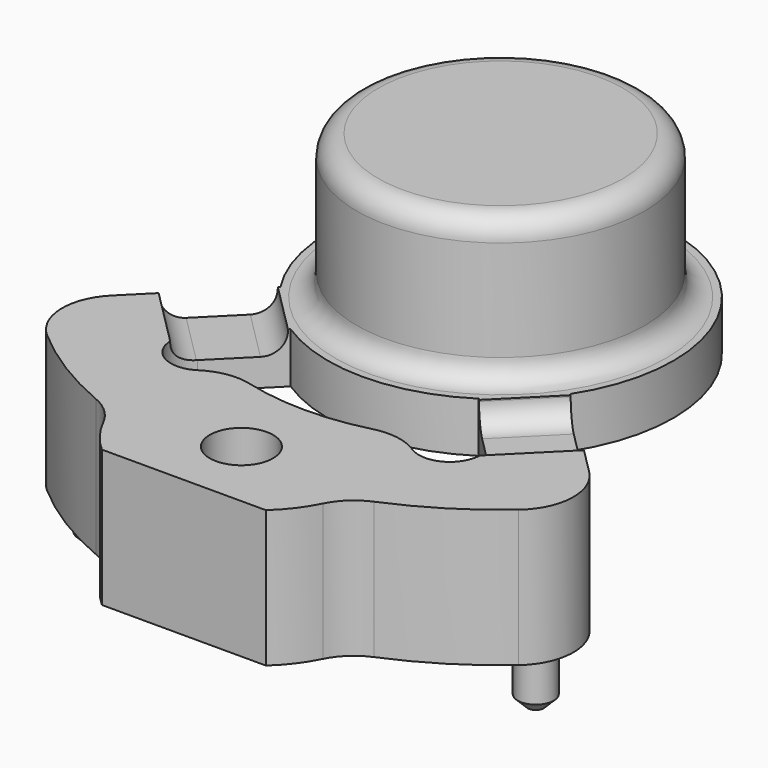
from build123d import *

# Parameters (mm, degrees)
F0_R      = 1.1
F1_DEPTH  = 4.75
F2_R      = 5
F3_DEPTH  = 5
F5_R      = 2
F7_DEPTH  = 0.8
F8_R      = 0.75
F9_R      = 9.5
F10_DEPTH = 3
F12_R     = 4.5172071506
F12_R_2   = 2.2672071506
F13_DEPTH = 3.7
F14_R     = 0.625
F15_DEPTH = 2
F16_SIZE  = 0.35


# Not quite as in the source:
# - a feature names something its author has since deleted; it is built from what else it names


with BuildPart() as f1:
    # F0 (on Top) → F1 (new body)
    with BuildSketch(Plane.XY):
        with BuildLine():
            Line((-5.0334316447, -3.2656646917), (-9.6784130262, -7.9106460732))
            ThreePointArc((-9.6784130262, -7.9106460732), (-7.1490584463, -10.2538267653), (-4.0757746589, -11.8168549509))
            ThreePointArc((-4.0757746589, -11.8168549509), (-3.593311946, -12.8676823003), (-2.8459674038, -13.75))
            Line((-2.8459674038, -13.75), (2.8459674038, -13.75))
            ThreePointArc((2.8459674038, -13.75), (3.593311946, -12.8676823003), (4.0757746589, -11.8168549509))
            ThreePointArc((4.0757746589, -11.8168549509), (7.1490584463, -10.2538267653), (9.6784130262, -7.9106460732))
            Line((9.6784130262, -7.9106460732), (5.0334316447, -3.2656646917))
            ThreePointArc((5.0334316447, -3.2656646917), (0, 6), (-5.0334316447, -3.2656646917))
        make_face()
        with Locations((0, -11.25)):
            Circle(F0_R, mode=Mode.SUBTRACT)
        with BuildLine():
            Line((-5.061459087, -6.82922604), (-3.2656646917, -5.0334316447))
            ThreePointArc((-3.2656646917, -5.0334316447), (0, -6), (3.2656646917, -5.0334316447))
            Line((3.2656646917, -5.0334316447), (5.061459087, -6.82922604))
            ThreePointArc((5.061459087, -6.82922604), (4.8326547168, -8.5179809488), (3.2656646917, -7.8480653995))
            ThreePointArc((3.2656646917, -7.8480653995), (0, -8.5003938964), (-3.2656646917, -7.8480653995))
            ThreePointArc((-3.2656646917, -7.8480653995), (-4.8326547168, -8.5179809488), (-5.061459087, -6.82922604))
        make_face(mode=Mode.SUBTRACT)
    extrude(amount=F1_DEPTH)

    # F2 (on face) → F3 (join)
    with BuildSketch(Plane.XY.offset(4.75)):
        Circle(F2_R)
    extrude(amount=F3_DEPTH)

    # F5
    f5_edges = [f1.edges().sort_by_distance(p)[0] for p in [
        (3.265665, -7.848065, 2.375),
        (-3.265665, -7.848065, 2.375),
        (-9.678413, -7.910646, 2.375),
        (-4.075775, -11.816855, 2.375),
        (9.678413, -7.910646, 2.375),
        (4.075775, -11.816855, 2.375),
    ]]
    fillet(f5_edges, radius=F5_R)

    # F6 (on face) → F7 (cut)
    with BuildSketch(Plane.XY.offset(4.75)):
        Polygon((4.3772207939, -8.619861481), (8.619861481, -4.3772207939), (6.2942457002, -2.1069760406), (2.0792905268, -6.3219312139), align=None)
        Polygon((-4.3772207939, -8.619861481), (-2.0792905268, -6.3219312139), (-6.2942457002, -2.1069760406), (-8.619861481, -4.3772207939), align=None)
    extrude(amount=-F7_DEPTH, mode=Mode.SUBTRACT)

    # F8
    f8_edges = [f1.edges().sort_by_distance(p)[0] for p in [
        (4.200611, -4.200611, 3.95),
        (-4.200611, -4.200611, 3.95),
        (-5, 0, 4.75),
        (-5, 0, 9.75),
        (6.378475, -6.618607, 3.95),
        (-6.378475, -6.618607, 3.95),
    ]]
    fillet(f8_edges, radius=F8_R)

    # F9 (on Top) → F10 (cut)
    with BuildSketch(Plane.XY):
        Circle(F9_R)
    extrude(amount=F10_DEPTH, mode=Mode.SUBTRACT)

    # F12 (on face) → F13 (cut)
    with BuildSketch(Plane(origin=(0, 0, 3), x_dir=(1, 0, 0), z_dir=(0, 0, -1))):
        Circle(F12_R)
        Circle(F12_R_2, mode=Mode.SUBTRACT)
    extrude(amount=-F13_DEPTH, mode=Mode.SUBTRACT)

    # F14 (on face) → F15 (join)
    with BuildSketch(Plane(origin=(0, 0, 0), x_dir=(1, 0, 0), z_dir=(0, 0, -1))):
        with Locations((7.6240489866, 8.007460935)):
            Circle(F14_R)
        with Locations((-7.6240489866, 8.007460935)):
            Circle(F14_R)
    extrude(amount=F15_DEPTH)

    # F16
    f16_edges = [f1.edges().sort_by_distance(p)[0] for p in [
        (6.999049, -8.007461, -2),
        (-8.249049, -8.007461, -2),
    ]]
    chamfer(f16_edges, length=F16_SIZE)


solid = f1.part
